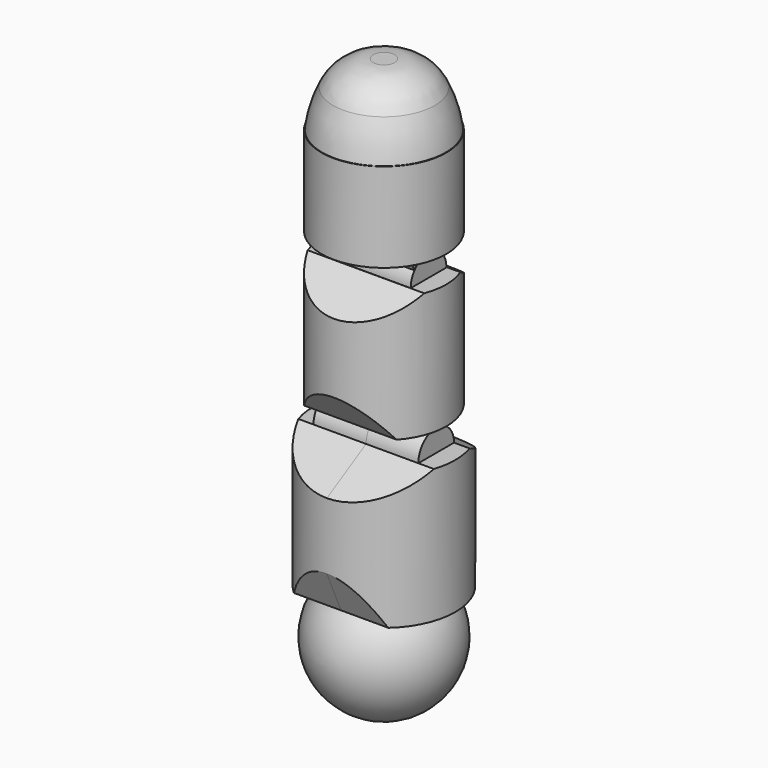
from build123d import *

# Parameters (mm, degrees)
F3_R           = 8
F4_DEPTH       = 15
F5_R           = 2.5
F6_DEPTH       = 5.85349
F6_DEPTH_BACK  = 5.90007
F8_DEPTH       = 25
F8_DEPTH_BACK  = 25
F10_DEPTH      = 4
F10_DEPTH_BACK = 4
F11_W          = 7
F11_H          = 14
F13_T4_DEPTH   = 25.4878140401
F13_T9_DEPTH   = 25.4878140401
F15_DEPTH      = 5
F15_DEPTH_BACK = 5
F17_DEPTH      = 25
F17_DEPTH_BACK = 25
F19_DEPTH      = 5
F19_DEPTH_BACK = 5
F20_W          = 7
F20_H          = 10
F24_W          = 10
F24_H          = 3
F25_DEPTH      = 25
F25_DEPTH_BACK = 25
F26_R          = 5
F27_T1_DEPTH   = 24.3777308897


# Not quite as in the source:
# - a fillet or chamfer that OpenCascade refuses, or shapes differently, is made with other operations: its cross-section is extruded or revolved along the edge and cut away or added


with BuildPart() as f1:
    # F0 (on Top) → F1 (revolve)
    with BuildSketch(Plane.XY):
        with BuildLine():
            Line((0, -7.5), (0, 7.5))
            ThreePointArc((0, 7.5), (-7.5, 0), (0, -7.5))
        make_face()
    revolve(axis=Axis((0, 0, 0), (0, -1, 0)))

    # F3 (on offset) → F4 (join)
    with BuildSketch(Plane.XY.offset(5)):
        Circle(F3_R)
    extrude(amount=F4_DEPTH)

    # F5 (on Right) → F6 (join, two sides)
    with BuildSketch(Plane.YZ) as f6_sk:
        with Locations((0, 20)):
            Circle(F5_R)
    extrude(amount=F6_DEPTH)
    extrude(f6_sk.sketch, amount=-F6_DEPTH_BACK)

    # F7 (on Right) → F8 (cut, two sides)
    with BuildSketch(Plane.YZ) as f8_sk:
        Polygon((9.1371238232, 20), (2.5, 20), (9.1371238232, 16.2389874458), align=None)
        Polygon((-9.1371238232, 16.2389874458), (-2.5, 20), (-9.1371238232, 20), align=None)
        Polygon((-9.1371238232, 11.9537818628), (-9.1371238232, 5), (-6, 5), align=None)
        Polygon((9.1371238232, 11.9537818628), (6, 5), (9.1371238232, 5), align=None)
    extrude(amount=-F8_DEPTH, mode=Mode.SUBTRACT)
    extrude(f8_sk.sketch, amount=F8_DEPTH_BACK, mode=Mode.SUBTRACT)


with BuildPart() as f10:
    # F9 (on Right) → F10 (new body, two sides)
    with BuildSketch(Plane.YZ) as f10_sk:
        with BuildLine():
            ThreePointArc((-2.6, 20), (0, 22.6000001084), (2.6, 20))
            Line((2.6, 20), (4, 20))
            ThreePointArc((4, 20), (0, 24.0000001084), (-4, 20))
            Line((-4, 20), (-2.6, 20))
        make_face()
    extrude(amount=F10_DEPTH)
    extrude(f10_sk.sketch, amount=-F10_DEPTH_BACK)

    # F11 (on Right) → F12 (revolve)
    with BuildSketch(Plane.YZ):
        with Locations((-3.5, 30)):
            Rectangle(F11_W, F11_H)
    revolve(axis=Axis((0, 0, 30), (0, 0, 1)))

    # F13: chamfer of 1.75 on 2 edges, made by hand


with BuildPart() as f13_tool2:
    # F13_s3 → F13_t4 (new body)
    with BuildSketch(Plane.YZ.offset(-12.74390702)):
        with BuildLine():
            Line((-1.4142136966, 20), (-2.5141576828, 23.1111110268))
            ThreePointArc((-2.5141576828, 23.1111110268), (-3.5976530662, 21.7483972072), (-4, 20))
            Line((-4, 20), (-1.4142136966, 20))
        make_face()
    extrude(amount=F13_T4_DEPTH)

    split(bisect_by=Plane.XY.offset(23), keep=Keep.BOTTOM)


with BuildPart() as f10_1:
    add(f10.part)

    # F13_t1: cut F13_tool2
    add(f13_tool2.part, mode=Mode.SUBTRACT)


with BuildPart() as f13_tool7:
    # F13_s8 → F13_t9 (new body)
    with BuildSketch(Plane.YZ.offset(12.74390702)):
        with BuildLine():
            Line((2.5141576828, 23.1111110268), (1.4142136966, 20))
            Line((1.4142136966, 20), (4, 20))
            ThreePointArc((4, 20), (3.5976530662, 21.7483972072), (2.5141576828, 23.1111110268))
        make_face()
    extrude(amount=-F13_T9_DEPTH)

    split(bisect_by=Plane.XY.offset(23), keep=Keep.BOTTOM)


with BuildPart() as f10_2:
    add(f10_1.part)

    # F13_t6: cut F13_tool7
    add(f13_tool7.part, mode=Mode.SUBTRACT)

    # F14 (on Right) → F15 (join, two sides)
    with BuildSketch(Plane.YZ) as f15_sk:
        with BuildLine():
            Line((-2.5, 37), (2.5, 37))
            ThreePointArc((2.5, 37), (0, 39.5), (-2.5, 37))
        make_face()
    extrude(amount=F15_DEPTH)
    extrude(f15_sk.sketch, amount=-F15_DEPTH_BACK)

    # F16 (on Right) → F17 (cut, two sides)
    with BuildSketch(Plane.YZ) as f17_sk:
        Polygon((-8.9805674515, 23), (-4.7004079688, 23), (-8.9805674515, 29.3250767589), align=None)
        Polygon((9.0322339683, 29.3250767589), (4.7520744856, 23), (9.0322339683, 23), align=None)
        Polygon((-8.9805674515, 32.9242510796), (-2.5218809023, 37), (-8.9805674515, 37), align=None)
        Polygon((9.0322339683, 37), (2.5735474192, 37), (9.0322339683, 32.9242510796), align=None)
    extrude(amount=-F17_DEPTH, mode=Mode.SUBTRACT)
    extrude(f17_sk.sketch, amount=F17_DEPTH_BACK, mode=Mode.SUBTRACT)


with BuildPart() as f19:
    # F18 (on Right) → F19 (new body, two sides)
    with BuildSketch(Plane.YZ) as f19_sk:
        with BuildLine():
            ThreePointArc((-2.55, 37), (0, 39.55), (2.55, 37))
            Line((2.55, 37), (3.55, 37))
            ThreePointArc((3.55, 37), (0, 40.55), (-3.55, 37))
            Line((-3.55, 37), (-2.55, 37))
        make_face()
    extrude(amount=F19_DEPTH)
    extrude(f19_sk.sketch, amount=-F19_DEPTH_BACK)

    # F20 (on Right) → F21 (revolve)
    with BuildSketch(Plane.YZ):
        with Locations((-3.5, 45)):
            Rectangle(F20_W, F20_H)
    revolve(axis=Axis((0, 0, 45), (0, 0, 1)))

    # F22 (on Right) → F23 (revolve)
    with BuildSketch(Plane.YZ):
        with BuildLine():
            Line((-6.9393450394, 50), (0, 50))
            Line((0, 50), (0, 60))
            ThreePointArc((0, 60), (-4.7123372957, 55.8623279649), (-6.9393450394, 50))
        make_face()
    revolve(axis=Axis((0, 0, 55), (0, 0, 1)))

    # F24 (on Right) → F25 (cut, two sides)
    with BuildSketch(Plane.YZ) as f25_sk:
        with Locations((0, 58.5)):
            Rectangle(F24_W, F24_H)
    extrude(amount=-F25_DEPTH, mode=Mode.SUBTRACT)
    extrude(f25_sk.sketch, amount=F25_DEPTH_BACK, mode=Mode.SUBTRACT)

    # F26
    f26_edges = [f19.edges().sort_by_distance(p)[0] for p in [
        (0, 3.825452, 57),
    ]]
    fillet(f26_edges, radius=F26_R)

    # F27: chamfer of 1.5 on 2 edges, made by hand

    # F27_s2 → F27_t1 (cut)
    with BuildSketch(Plane.YZ.offset(-12.1888654448)):
        with BuildLine():
            Line((-2.4197472963, 39.5975609756), (-1.3973188612, 37))
            Line((-1.3973188612, 37), (-3.55, 37))
            ThreePointArc((-3.55, 37), (-3.2459574924, 38.4374491147), (-2.4197472963, 39.5975609756))
        make_face()
        with BuildLine():
            Line((2.4197472963, 39.5975609756), (1.3973188612, 37))
            Line((1.3973188612, 37), (3.55, 37))
            ThreePointArc((3.55, 37), (3.2459574924, 38.4374491147), (2.4197472963, 39.5975609756))
        make_face()
    extrude(amount=F27_T1_DEPTH, mode=Mode.SUBTRACT)


solid = Compound([f1.part, f10_2.part, f19.part])
